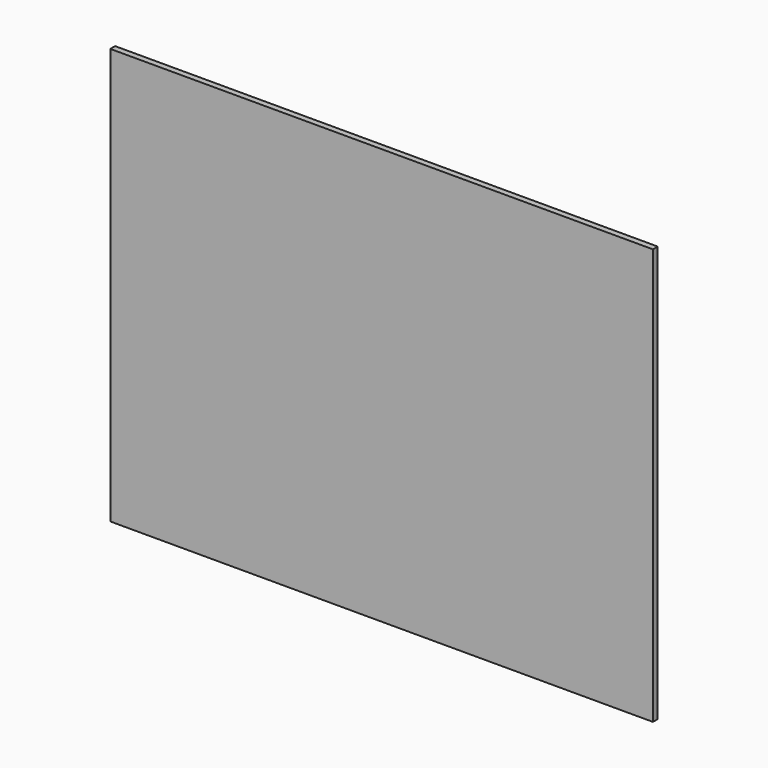
from build123d import *

# Parameters (mm, degrees)
F0_W     = 45.72
F0_H     = 35.052
F2_DEPTH = 0.508


# Not quite as in the source:
# - the program builds the solid bodies; features that only make, move or delete a surface that nothing else refers to are left out


with BuildPart() as f2:
    # F0 (on Front) → F2 (new body)
    with BuildSketch(Plane.XZ):
        with Locations((-40.2947817915, -17.526)):
            Rectangle(F0_W, F0_H)
    extrude(amount=-F2_DEPTH)


solid = f2.part
